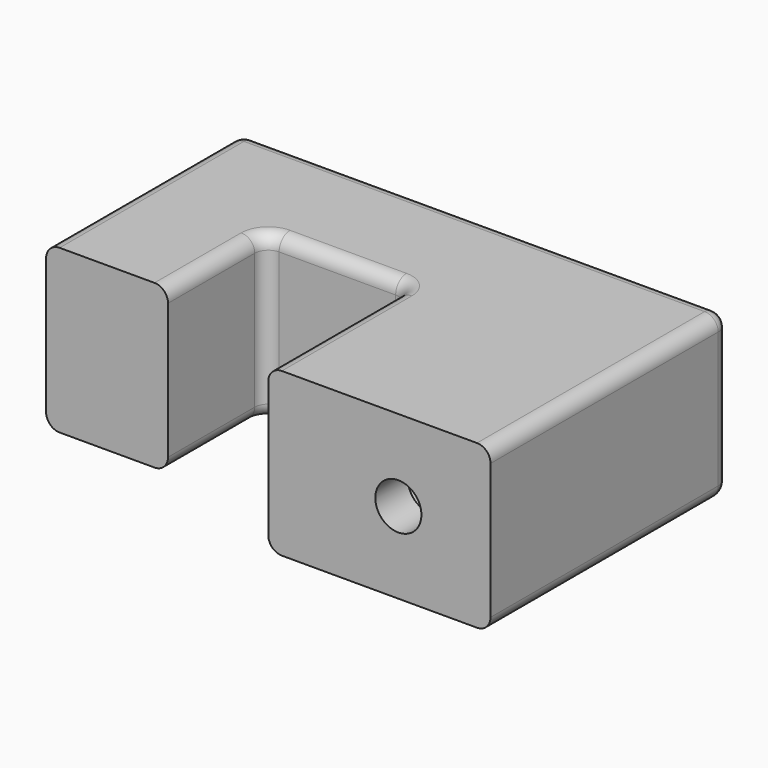
from build123d import *

# Parameters (mm, degrees)
F1_DEPTH = 15.24
F2_R     = 2.159
F3_DEPTH = 27.94
F4_R     = 3.683
F5_DEPTH = 24.13
F6_F1_R  = 1.27
F6_F2_R  = 1.27
F6_F3_R  = 1.27


with BuildPart() as f1:
    # F0 (on Top) → F1 (new body)
    with BuildSketch(Plane.XY):
        Polygon((-11.43, 0), (0, 0), (0, 11.43), (13.462, 11.43), (13.462, -5.08), (34.29, -5.08), (34.29, 22.86), (-11.43, 22.86), align=None)
    extrude(amount=F1_DEPTH)

    # F2 (on face) → F3 (cut, through all)
    with BuildSketch(Plane.XZ.offset(5.08)):
        with Locations((25.654, 7.62)):
            Circle(F2_R)
    extrude(amount=-F3_DEPTH, mode=Mode.SUBTRACT)

    # F4 (on face) → F5 (cut)
    with BuildSketch(Plane(origin=(0, 22.86, 0), x_dir=(-1, 0, 0), z_dir=(0, 1, 0))):
        with Locations((-25.654, 7.62)):
            Circle(F4_R)
    extrude(amount=-F5_DEPTH, mode=Mode.SUBTRACT)

    # F6: fillet of radius 1.27 on 14 edges, made by hand

    # F6_f1
    f6_f1_edges = [f1.edges().sort_by_distance(p)[0] for p in [
        (0, 11.43, 7.62),
        (13.462, 11.43, 7.62),
    ]]
    fillet(f6_f1_edges, radius=F6_F1_R)

    # F6_f2
    f6_f2_edges = [f1.edges().sort_by_distance(p)[0] for p in [
        (6.731, 11.43, 15.24),
        (-11.43, 22.86, 7.62),
        (-11.43, 11.43, 15.24),
        (-11.43, 11.43, 0),
        (11.43, 22.86, 15.24),
        (34.29, 22.86, 7.62),
        (34.29, 8.89, 15.24),
        (34.29, 8.89, 0),
        (11.43, 22.86, 0),
        (29.337, 22.86, 7.62),
        (0.3719743879, 11.0580256121, 15.24),
        (13.0900256121, 11.0580256121, 15.24),
    ]]
    fillet(f6_f2_edges, radius=F6_F2_R)

    # F6_f3
    f6_f3_edges = [f1.edges().sort_by_distance(p)[0] for p in [
        (0, 5.08, 0),
        (6.731, 11.43, 0),
        (0.3719743879, 11.0580256121, 0),
        (13.0900256121, 11.0580256121, 0),
    ]]
    fillet(f6_f3_edges, radius=F6_F3_R)


solid = f1.part
